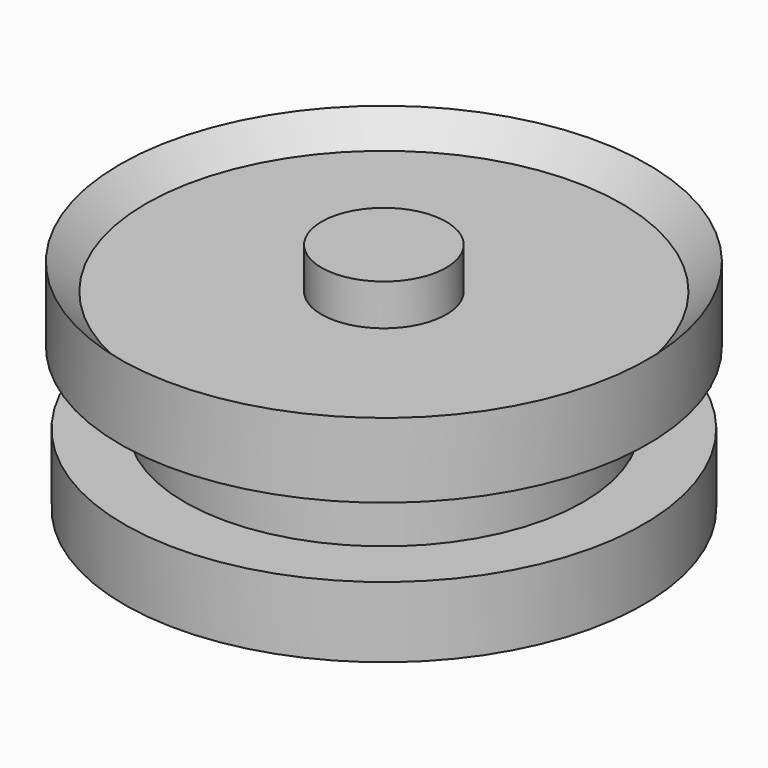
from build123d import *


# Not quite as in the source:
# - a fillet or chamfer that OpenCascade refuses, or shapes differently, is made with other operations: its cross-section is extruded or revolved along the edge and cut away or added


with BuildPart() as f1:
    # F0 (on Front) → F1 (revolve)
    with BuildSketch(Plane.XZ):
        Polygon((0, 2.4378150702), (0, 2.7715591714), (0, 9.970895946), (-2.0202985033, 9.970895946), (-2.0202985033, 8.6359195411), (-6.4543271437, 8.6359195411), (-6.4543271437, 9.9232187495), (-8.5521470755, 9.9232187495), (-8.5521470755, 7.0625548251), (-6.4543271437, 7.0625548251), (-6.4543271437, 4.7263461165), (-8.4091145545, 4.7263461165), (-8.4091145545, 2.4378150702), align=None)
    revolve(axis=Axis((0, 0, 6.3712275587), (0, 0, 1)))

    # F2: chamfer of 2.54 on 1 edges, made by hand


with BuildPart() as f2_tool2:
    # F2_s3 → F2_t4 (revolve)
    with BuildSketch(Plane.XZ):
        Polygon((-6.4543271437, 7.3832187495), (-8.9943271437, 9.9232187495), (-6.4543271437, 9.9232187495), align=None)
    revolve(axis=Axis((0, 0, 9.9232187495), (0, 0, 1)))

    split(bisect_by=Plane.XY.offset(8.6359195411), keep=Keep.TOP)


with BuildPart() as f1_1:
    add(f1.part)

    # F2_t1: cut F2_tool2
    add(f2_tool2.part, mode=Mode.SUBTRACT)


solid = f1_1.part
